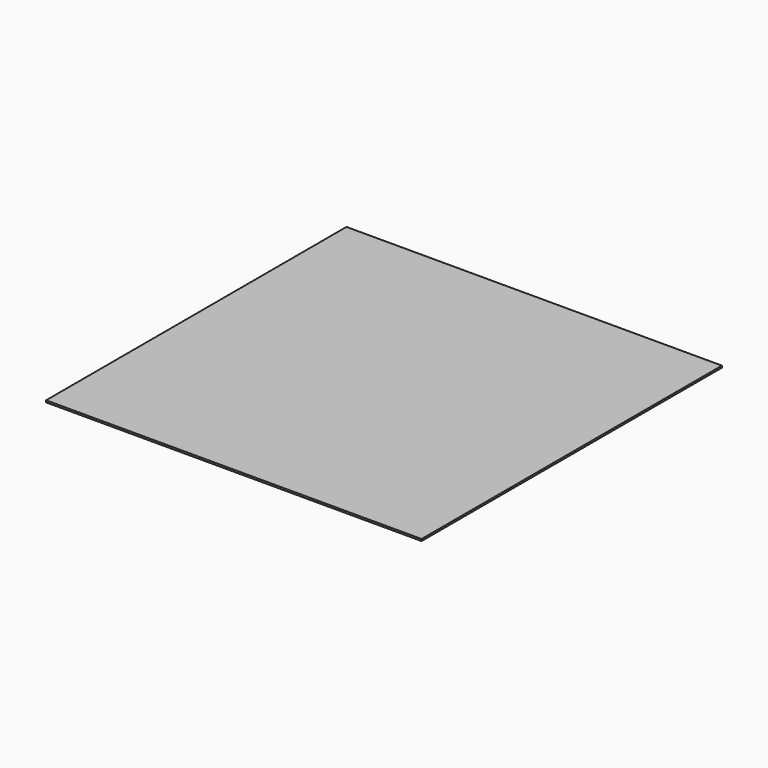
from build123d import *

# Parameters (mm, degrees)
F1_DEPTH = 50


# Not quite as in the source:
# - the program builds the solid bodies; features that only make, move or delete a surface that nothing else refers to are left out


with BuildPart() as f1:
    # F0 (on Top) → F1 (new body)
    with BuildSketch(Plane.XY):
        Polygon((5000, 5000), (-5000, 5000), (-5000, 0), (-2000, 0), (5000, 0), align=None)
        Polygon((-2000, 0), (-5000, 0), (-5000, -5000), (5000, -5000), (5000, 0), align=None)
    extrude(amount=-F1_DEPTH)


solid = f1.part
